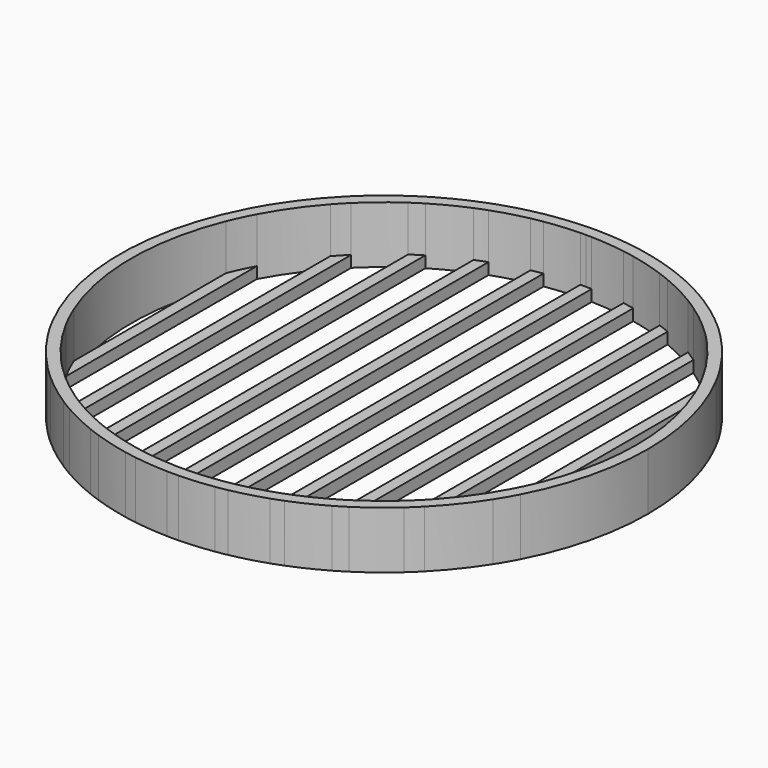
from build123d import *

# Parameters (mm, degrees)
F1_DEPTH = 10
F2_DEPTH = 2


with BuildPart() as f1:
    # F0 (on Top) → F1 (new body)
    with BuildSketch(Plane.XY):
        with BuildLine():
            ThreePointArc((41, 16.6451945017), (43.4299004143, 8.4797553031), (44.25, 0))
            ThreePointArc((44.25, 0), (43.4299004143, -8.4797553031), (41, -16.6451945017))
            Line((41, -16.6451945017), (41, -21.4023947258))
            ThreePointArc((41, -21.4023947258), (44.9183286644, -11.0184504355), (46.25, 0))
            ThreePointArc((46.25, 0), (44.9183286644, 11.0184504355), (41, 21.4023947258))
            Line((41, 21.4023947258), (41, 16.6451945017))
        make_face()
        with BuildLine():
            ThreePointArc((39, 20.9060397972), (40.0566935812, 18.8022285738), (41, 16.6451945017))
            Line((41, 16.6451945017), (41, 21.4023947258))
            ThreePointArc((41, 21.4023947258), (40.037360682, 23.153234107), (39, 24.8608628169))
            Line((39, 24.8608628169), (39, 20.9060397972))
        make_face()
        with BuildLine():
            Line((41, -21.4023947258), (41, -16.6451945017))
            ThreePointArc((41, -16.6451945017), (40.0566935812, -18.8022285738), (39, -20.9060397972))
            Line((39, -20.9060397972), (39, -24.8608628169))
            ThreePointArc((39, -24.8608628169), (40.037360682, -23.153234107), (41, -21.4023947258))
        make_face()
        with BuildLine():
            ThreePointArc((33, 29.4798660106), (36.2543462772, 25.3709455089), (39, 20.9060397972))
            Line((39, 20.9060397972), (39, 24.8608628169))
            ThreePointArc((39, 24.8608628169), (36.1970613266, 28.7894989765), (33, 32.4046678736))
            Line((33, 32.4046678736), (33, 29.4798660106))
        make_face()
        with BuildLine():
            Line((39, -24.8608628169), (39, -20.9060397972))
            ThreePointArc((39, -20.9060397972), (36.2543462772, -25.3709455089), (33, -29.4798660106))
            Line((33, -29.4798660106), (33, -32.4046678736))
            ThreePointArc((33, -32.4046678736), (36.1970613266, -28.7894989765), (39, -24.8608628169))
        make_face()
        with BuildLine():
            ThreePointArc((31, 31.5762964896), (32.0171634469, 30.544455222), (33, 29.4798660106))
            Line((33, 29.4798660106), (33, 32.4046678736))
            ThreePointArc((33, 32.4046678736), (32.0143704935, 33.3787744219), (31, 34.322915086))
            Line((31, 34.322915086), (31, 31.5762964896))
        make_face()
        with BuildLine():
            Line((33, -32.4046678736), (33, -29.4798660106))
            ThreePointArc((33, -29.4798660106), (32.0171634469, -30.544455222), (31, -31.5762964896))
            Line((31, -31.5762964896), (31, -34.322915086))
            ThreePointArc((31, -34.322915086), (32.0143704935, -33.3787744219), (33, -32.4046678736))
        make_face()
        with BuildLine():
            ThreePointArc((25, 36.5111284405), (28.10850657, 34.175639839), (31, 31.5762964896))
            Line((31, 31.5762964896), (31, 34.322915086))
            ThreePointArc((31, 34.322915086), (28.0938165786, 36.7396239781), (25, 38.9109560407))
            Line((25, 38.9109560407), (25, 36.5111284405))
        make_face()
        with BuildLine():
            Line((31, -34.322915086), (31, -31.5762964896))
            ThreePointArc((31, -31.5762964896), (28.10850657, -34.175639839), (25, -36.5111284405))
            Line((25, -36.5111284405), (25, -38.9109560407))
            ThreePointArc((25, -38.9109560407), (28.0938165786, -36.7396239781), (31, -34.322915086))
        make_face()
        with BuildLine():
            ThreePointArc((23, 37.8029430071), (24.0086900146, 37.1704896898), (25, 36.5111284405))
            Line((25, 36.5111284405), (25, 38.9109560407))
            ThreePointArc((25, 38.9109560407), (24.0076827356, 39.5309204252), (23, 40.1255841079))
            Line((23, 40.1255841079), (23, 37.8029430071))
        make_face()
        with BuildLine():
            Line((25, -38.9109560407), (25, -36.5111284405))
            ThreePointArc((25, -36.5111284405), (24.0086900146, -37.1704896898), (23, -37.8029430071))
            Line((23, -37.8029430071), (23, -40.1255841079))
            ThreePointArc((23, -40.1255841079), (24.0076827356, -39.5309204252), (25, -38.9109560407))
        make_face()
        with BuildLine():
            ThreePointArc((17, 40.8541613548), (20.0581026857, 39.4428069063), (23, 37.8029430071))
            Line((23, 37.8029430071), (23, 40.1255841079))
            ThreePointArc((23, 40.1255841079), (20.0520163196, 41.6770817299), (17, 43.0123528768))
            Line((17, 43.0123528768), (17, 40.8541613548))
        make_face()
        with BuildLine():
            Line((23, -40.1255841079), (23, -37.8029430071))
            ThreePointArc((23, -37.8029430071), (20.0581026857, -39.4428069063), (17, -40.8541613548))
            Line((17, -40.8541613548), (17, -43.0123528768))
            ThreePointArc((17, -43.0123528768), (20.0520163196, -41.6770817299), (23, -40.1255841079))
        make_face()
        with BuildLine():
            ThreePointArc((15, 41.6300672591), (16.0047026681, 41.2542360553), (17, 40.8541613548))
            Line((17, 40.8541613548), (17, 43.0123528768))
            ThreePointArc((17, 43.0123528768), (16.0042503986, 43.392700644), (15, 43.75))
            Line((15, 43.75), (15, 41.6300672591))
        make_face()
        with BuildLine():
            Line((17, -43.0123528768), (17, -40.8541613548))
            ThreePointArc((17, -40.8541613548), (16.0047026681, -41.2542360553), (15, -41.6300672591))
            Line((15, -41.6300672591), (15, -43.75))
            ThreePointArc((15, -43.75), (16.0042503986, -43.392700644), (17, -43.0123528768))
        make_face()
        with BuildLine():
            ThreePointArc((9, 43.3250793421), (12.0298905436, 42.5833797803), (15, 41.6300672591))
            Line((15, 41.6300672591), (15, 43.75))
            ThreePointArc((15, 43.75), (12.0271676626, 44.6588147852), (9, 45.3658737379))
            Line((9, 45.3658737379), (9, 43.3250793421))
        make_face()
        with BuildLine():
            Line((15, -43.75), (15, -41.6300672591))
            ThreePointArc((15, -41.6300672591), (12.0298905436, -42.5833797803), (9, -43.3250793421))
            Line((9, -43.3250793421), (9, -45.3658737379))
            ThreePointArc((9, -45.3658737379), (12.0271676626, -44.6588147852), (15, -43.75))
        make_face()
        with BuildLine():
            ThreePointArc((7, 43.6928197763), (8.0021127371, 43.5204399305), (9, 43.3250793421))
            Line((9, 43.3250793421), (9, 45.3658737379))
            ThreePointArc((9, 45.3658737379), (8.0019283785, 45.5525152129), (7, 45.7172013579))
            Line((7, 45.7172013579), (7, 43.6928197763))
        make_face()
        with BuildLine():
            Line((9, -45.3658737379), (9, -43.3250793421))
            ThreePointArc((9, -43.3250793421), (8.0021127371, -43.5204399305), (7, -43.6928197763))
            Line((7, -43.6928197763), (7, -45.7172013579))
            ThreePointArc((7, -45.7172013579), (8.0019283785, -45.5525152129), (9, -45.3658737379))
        make_face()
        with BuildLine():
            ThreePointArc((1, 44.2386991219), (4.0093011941, 44.0679929647), (7, 43.6928197763))
            Line((7, 43.6928197763), (7, 45.7172013579))
            ThreePointArc((7, 45.7172013579), (4.0085056435, 46.075963175), (1, 46.2391879254))
            Line((1, 46.2391879254), (1, 44.2386991219))
        make_face()
        with BuildLine():
            Line((7, -45.7172013579), (7, -43.6928197763))
            ThreePointArc((7, -43.6928197763), (4.0093011941, -44.0679929647), (1, -44.2386991219))
            Line((1, -44.2386991219), (1, -46.2391879254))
            ThreePointArc((1, -46.2391879254), (4.0085056435, -46.075963175), (7, -45.7172013579))
        make_face()
        with BuildLine():
            ThreePointArc((0, 44.25), (0.5000319264, 44.2471746903), (1, 44.2386991219))
            Line((1, 44.2386991219), (1, 46.2391879254))
            ThreePointArc((1, 46.2391879254), (0, 46.25), (-1, 46.2391879254))
            Line((-1, 46.2391879254), (-1, 44.2386991219))
            ThreePointArc((-1, 44.2386991219), (-0.5000319264, 44.2471746903), (0, 44.25))
        make_face()
        with BuildLine():
            Line((1, -46.2391879254), (1, -44.2386991219))
            ThreePointArc((1, -44.2386991219), (0.5000319264, -44.2471746903), (0, -44.25))
            ThreePointArc((0, -44.25), (-0.5000319264, -44.2471746903), (-1, -44.2386991219))
            Line((-1, -44.2386991219), (-1, -46.2391879254))
            ThreePointArc((-1, -46.2391879254), (0, -46.25), (1, -46.2391879254))
        make_face()
        with BuildLine():
            ThreePointArc((-7, 43.6928197763), (-4.0093011941, 44.0679929647), (-1, 44.2386991219))
            Line((-1, 44.2386991219), (-1, 46.2391879254))
            ThreePointArc((-1, 46.2391879254), (-4.0085056435, 46.075963175), (-7, 45.7172013579))
            Line((-7, 45.7172013579), (-7, 43.6928197763))
        make_face()
        with BuildLine():
            Line((-1, -46.2391879254), (-1, -44.2386991219))
            ThreePointArc((-1, -44.2386991219), (-4.0093011941, -44.0679929647), (-7, -43.6928197763))
            Line((-7, -43.6928197763), (-7, -45.7172013579))
            ThreePointArc((-7, -45.7172013579), (-4.0085056435, -46.075963175), (-1, -46.2391879254))
        make_face()
        with BuildLine():
            ThreePointArc((-9, 43.3250793421), (-8.0021127371, 43.5204399305), (-7, 43.6928197763))
            Line((-7, 43.6928197763), (-7, 45.7172013579))
            ThreePointArc((-7, 45.7172013579), (-8.0019283785, 45.5525152129), (-9, 45.3658737379))
            Line((-9, 45.3658737379), (-9, 43.3250793421))
        make_face()
        with BuildLine():
            Line((-7, -45.7172013579), (-7, -43.6928197763))
            ThreePointArc((-7, -43.6928197763), (-8.0021127371, -43.5204399305), (-9, -43.3250793421))
            Line((-9, -43.3250793421), (-9, -45.3658737379))
            ThreePointArc((-9, -45.3658737379), (-8.0019283785, -45.5525152129), (-7, -45.7172013579))
        make_face()
        with BuildLine():
            ThreePointArc((-15, 41.6300672591), (-12.0298905436, 42.5833797803), (-9, 43.3250793421))
            Line((-9, 43.3250793421), (-9, 45.3658737379))
            ThreePointArc((-9, 45.3658737379), (-12.0271676626, 44.6588147852), (-15, 43.75))
            Line((-15, 43.75), (-15, 41.6300672591))
        make_face()
        with BuildLine():
            Line((-9, -45.3658737379), (-9, -43.3250793421))
            ThreePointArc((-9, -43.3250793421), (-12.0298905436, -42.5833797803), (-15, -41.6300672591))
            Line((-15, -41.6300672591), (-15, -43.75))
            ThreePointArc((-15, -43.75), (-12.0271676626, -44.6588147852), (-9, -45.3658737379))
        make_face()
        with BuildLine():
            ThreePointArc((-17, 40.8541613548), (-16.0047026681, 41.2542360553), (-15, 41.6300672591))
            Line((-15, 41.6300672591), (-15, 43.75))
            ThreePointArc((-15, 43.75), (-16.0042503986, 43.392700644), (-17, 43.0123528768))
            Line((-17, 43.0123528768), (-17, 40.8541613548))
        make_face()
        with BuildLine():
            Line((-15, -43.75), (-15, -41.6300672591))
            ThreePointArc((-15, -41.6300672591), (-16.0047026681, -41.2542360553), (-17, -40.8541613548))
            Line((-17, -40.8541613548), (-17, -43.0123528768))
            ThreePointArc((-17, -43.0123528768), (-16.0042503986, -43.392700644), (-15, -43.75))
        make_face()
        with BuildLine():
            ThreePointArc((-23, 37.8029430071), (-20.0581026857, 39.4428069063), (-17, 40.8541613548))
            Line((-17, 40.8541613548), (-17, 43.0123528768))
            ThreePointArc((-17, 43.0123528768), (-20.0520163196, 41.6770817299), (-23, 40.1255841079))
            Line((-23, 40.1255841079), (-23, 37.8029430071))
        make_face()
        with BuildLine():
            Line((-17, -43.0123528768), (-17, -40.8541613548))
            ThreePointArc((-17, -40.8541613548), (-20.0581026857, -39.4428069063), (-23, -37.8029430071))
            Line((-23, -37.8029430071), (-23, -40.1255841079))
            ThreePointArc((-23, -40.1255841079), (-20.0520163196, -41.6770817299), (-17, -43.0123528768))
        make_face()
        with BuildLine():
            ThreePointArc((-25, 36.5111284405), (-24.0086900146, 37.1704896898), (-23, 37.8029430071))
            Line((-23, 37.8029430071), (-23, 40.1255841079))
            ThreePointArc((-23, 40.1255841079), (-24.0076827356, 39.5309204252), (-25, 38.9109560407))
            Line((-25, 38.9109560407), (-25, 36.5111284405))
        make_face()
        with BuildLine():
            Line((-23, -40.1255841079), (-23, -37.8029430071))
            ThreePointArc((-23, -37.8029430071), (-24.0086900146, -37.1704896898), (-25, -36.5111284405))
            Line((-25, -36.5111284405), (-25, -38.9109560407))
            ThreePointArc((-25, -38.9109560407), (-24.0076827356, -39.5309204252), (-23, -40.1255841079))
        make_face()
        with BuildLine():
            ThreePointArc((-31, 31.5762964896), (-28.10850657, 34.175639839), (-25, 36.5111284405))
            Line((-25, 36.5111284405), (-25, 38.9109560407))
            ThreePointArc((-25, 38.9109560407), (-28.0938165786, 36.7396239781), (-31, 34.322915086))
            Line((-31, 34.322915086), (-31, 31.5762964896))
        make_face()
        with BuildLine():
            Line((-25, -38.9109560407), (-25, -36.5111284405))
            ThreePointArc((-25, -36.5111284405), (-28.10850657, -34.175639839), (-31, -31.5762964896))
            Line((-31, -31.5762964896), (-31, -34.322915086))
            ThreePointArc((-31, -34.322915086), (-28.0938165786, -36.7396239781), (-25, -38.9109560407))
        make_face()
        with BuildLine():
            ThreePointArc((-33, 29.4798660105), (-32.0171634469, 30.544455222), (-31, 31.5762964896))
            Line((-31, 31.5762964896), (-31, 34.322915086))
            ThreePointArc((-31, 34.322915086), (-32.0143704935, 33.3787744219), (-33, 32.4046678736))
            Line((-33, 32.4046678736), (-33, 29.4798660105))
        make_face()
        with BuildLine():
            Line((-31, -34.322915086), (-31, -31.5762964896))
            ThreePointArc((-31, -31.5762964896), (-32.0171634469, -30.544455222), (-33, -29.4798660105))
            Line((-33, -29.4798660105), (-33, -32.4046678736))
            ThreePointArc((-33, -32.4046678736), (-32.0143704935, -33.3787744219), (-31, -34.322915086))
        make_face()
        with BuildLine():
            ThreePointArc((-39, 20.9060397972), (-36.2543462772, 25.3709455089), (-33, 29.4798660105))
            Line((-33, 29.4798660105), (-33, 32.4046678736))
            ThreePointArc((-33, 32.4046678736), (-36.1970613266, 28.7894989765), (-39, 24.8608628169))
            Line((-39, 24.8608628169), (-39, 20.9060397972))
        make_face()
        with BuildLine():
            Line((-33, -32.4046678736), (-33, -29.4798660105))
            ThreePointArc((-33, -29.4798660105), (-36.2543462772, -25.3709455089), (-39, -20.9060397972))
            Line((-39, -20.9060397972), (-39, -24.8608628169))
            ThreePointArc((-39, -24.8608628169), (-36.1970613266, -28.7894989765), (-33, -32.4046678736))
        make_face()
        with BuildLine():
            ThreePointArc((-41, 16.6451945017), (-40.0566935812, 18.8022285738), (-39, 20.9060397972))
            Line((-39, 20.9060397972), (-39, 24.8608628169))
            ThreePointArc((-39, 24.8608628169), (-40.037360682, 23.153234107), (-41, 21.4023947258))
            Line((-41, 21.4023947258), (-41, 16.6451945017))
        make_face()
        with BuildLine():
            Line((-39, -24.8608628169), (-39, -20.9060397972))
            ThreePointArc((-39, -20.9060397972), (-40.0566935812, -18.8022285738), (-41, -16.6451945017))
            Line((-41, -16.6451945017), (-41, -21.4023947258))
            ThreePointArc((-41, -21.4023947258), (-40.037360682, -23.153234107), (-39, -24.8608628169))
        make_face()
        with BuildLine():
            ThreePointArc((-41, -16.6451945017), (-44.25, 0), (-41, 16.6451945017))
            Line((-41, 16.6451945017), (-41, 21.4023947258))
            ThreePointArc((-41, 21.4023947258), (-46.25, 0), (-41, -21.4023947258))
            Line((-41, -21.4023947258), (-41, -16.6451945017))
        make_face()
    extrude(amount=F1_DEPTH)

    # F0 (on Top) → F2 (join)
    with BuildSketch(Plane.XY):
        with BuildLine():
            Line((-31, -31.5762964896), (-31, 31.5762964896))
            ThreePointArc((-31, 31.5762964896), (-32.0171634469, 30.544455222), (-33, 29.4798660105))
            Line((-33, 29.4798660105), (-33, -29.4798660105))
            ThreePointArc((-33, -29.4798660105), (-32.0171634469, -30.544455222), (-31, -31.5762964896))
        make_face()
        with BuildLine():
            Line((-23, -37.8029430071), (-23, 37.8029430071))
            ThreePointArc((-23, 37.8029430071), (-24.0086900146, 37.1704896898), (-25, 36.5111284405))
            Line((-25, 36.5111284405), (-25, -36.5111284405))
            ThreePointArc((-25, -36.5111284405), (-24.0086900146, -37.1704896898), (-23, -37.8029430071))
        make_face()
        with BuildLine():
            Line((-15, -41.6300672591), (-15, 41.6300672591))
            ThreePointArc((-15, 41.6300672591), (-16.0047026681, 41.2542360553), (-17, 40.8541613548))
            Line((-17, 40.8541613548), (-17, -40.8541613548))
            ThreePointArc((-17, -40.8541613548), (-16.0047026681, -41.2542360553), (-15, -41.6300672591))
        make_face()
        with BuildLine():
            Line((-7, -43.6928197763), (-7, 43.6928197763))
            ThreePointArc((-7, 43.6928197763), (-8.0021127371, 43.5204399305), (-9, 43.3250793421))
            Line((-9, 43.3250793421), (-9, -43.3250793421))
            ThreePointArc((-9, -43.3250793421), (-8.0021127371, -43.5204399305), (-7, -43.6928197763))
        make_face()
        with BuildLine():
            Line((0, -44.25), (0, 44.25))
            ThreePointArc((0, 44.25), (-0.5000319264, 44.2471746903), (-1, 44.2386991219))
            Line((-1, 44.2386991219), (-1, -44.2386991219))
            ThreePointArc((-1, -44.2386991219), (-0.5000319264, -44.2471746903), (0, -44.25))
        make_face()
        with BuildLine():
            Line((9, -43.3250793421), (9, 43.3250793421))
            ThreePointArc((9, 43.3250793421), (8.0021127371, 43.5204399305), (7, 43.6928197763))
            Line((7, 43.6928197763), (7, -43.6928197763))
            ThreePointArc((7, -43.6928197763), (8.0021127371, -43.5204399305), (9, -43.3250793421))
        make_face()
        with BuildLine():
            Line((17, -40.8541613548), (17, 40.8541613548))
            ThreePointArc((17, 40.8541613548), (16.0047026681, 41.2542360553), (15, 41.6300672591))
            Line((15, 41.6300672591), (15, -41.6300672591))
            ThreePointArc((15, -41.6300672591), (16.0047026681, -41.2542360553), (17, -40.8541613548))
        make_face()
        with BuildLine():
            Line((25, -36.5111284405), (25, 36.5111284405))
            ThreePointArc((25, 36.5111284405), (24.0086900146, 37.1704896898), (23, 37.8029430071))
            Line((23, 37.8029430071), (23, -37.8029430071))
            ThreePointArc((23, -37.8029430071), (24.0086900146, -37.1704896898), (25, -36.5111284405))
        make_face()
        with BuildLine():
            Line((33, -29.4798660106), (33, 29.4798660106))
            ThreePointArc((33, 29.4798660106), (32.0171634469, 30.544455222), (31, 31.5762964896))
            Line((31, 31.5762964896), (31, -31.5762964896))
            ThreePointArc((31, -31.5762964896), (32.0171634469, -30.544455222), (33, -29.4798660106))
        make_face()
        with BuildLine():
            Line((41, -16.6451945017), (41, 16.6451945017))
            ThreePointArc((41, 16.6451945017), (40.0566935812, 18.8022285738), (39, 20.9060397972))
            Line((39, 20.9060397972), (39, -20.9060397972))
            ThreePointArc((39, -20.9060397972), (40.0566935812, -18.8022285738), (41, -16.6451945017))
        make_face()
        with BuildLine():
            Line((1, 38.2362119853), (1, 44.2386991219))
            ThreePointArc((1, 44.2386991219), (0.5000319264, 44.2471746903), (0, 44.25))
            Line((0, 44.25), (0, -44.25))
            ThreePointArc((0, -44.25), (0.5000319264, -44.2471746903), (1, -44.2386991219))
            Line((1, -44.2386991219), (1, 38.2362119853))
        make_face()
        with BuildLine():
            Line((-39, -20.9060397972), (-39, 20.9060397972))
            ThreePointArc((-39, 20.9060397972), (-40.0566935812, 18.8022285738), (-41, 16.6451945017))
            Line((-41, 16.6451945017), (-41, -16.6451945017))
            ThreePointArc((-41, -16.6451945017), (-40.0566935812, -18.8022285738), (-39, -20.9060397972))
        make_face()
    extrude(amount=F2_DEPTH)


solid = f1.part
